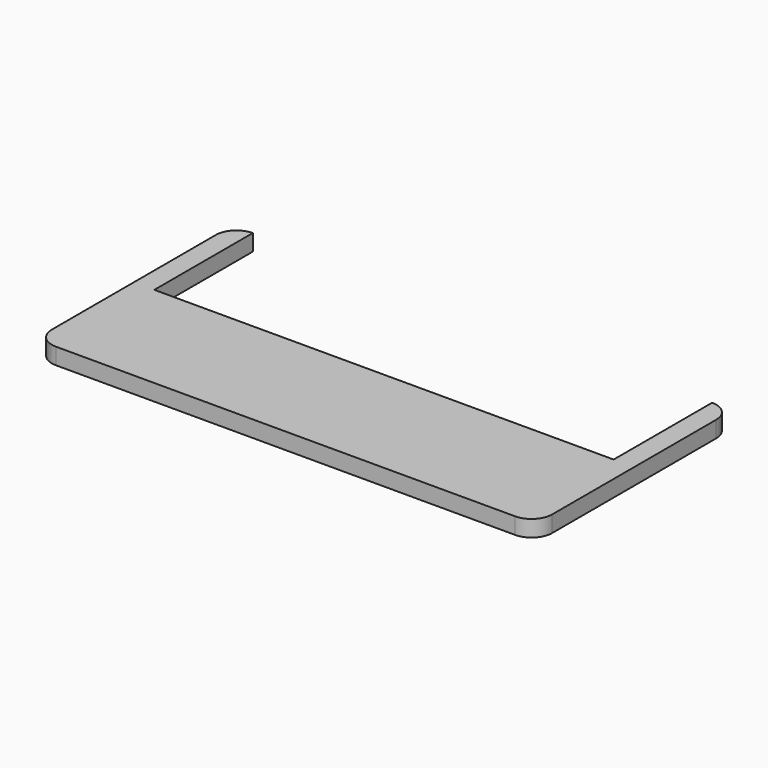
from build123d import *

# Parameters (mm, degrees)
F0_W     = 112
F0_H     = 30
F1_DEPTH = 4
F2_R     = 4.99999


# Not quite as in the source:
# - a fillet or chamfer is up to 0.001 mm smaller than in the source, because OpenCascade refuses the exact size


with BuildPart() as f1:
    # F0 (on Top) → F1 (new body)
    with BuildSketch(Plane.XY):
        with Locations((0, -15)):
            Rectangle(F0_W, F0_H)
        Polygon((-56, -30), (-56, 0), (-56, 30), (-61, 30), (-61, -30), align=None)
        Polygon((56, 30), (56, 0), (56, -30), (61, -30), (61, 30), align=None)
    extrude(amount=F1_DEPTH)

    # F2 (radius 5 in the source; OpenCascade refuses exactly that, so slightly less here)
    f2_edges = [f1.edges().sort_by_distance(p)[0] for p in [
        (-61, -30, 2),
        (61, -30, 2),
        (61, 30, 2),
        (-61, 30, 2),
    ]]
    fillet(f2_edges, radius=F2_R)


solid = f1.part
